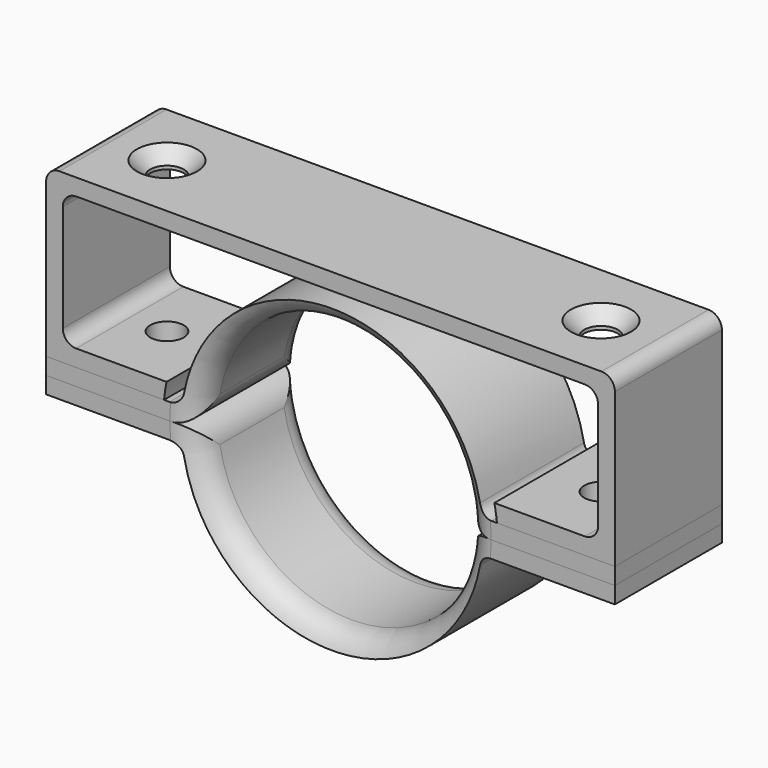
from build123d import *

# Parameters (mm, degrees)
F1_DEPTH      = 25.4
F2_DEPTH      = 25.4
F4_T1_DEPTH   = 48.6684264907
F4_T4_ANGLE   = 237.3879219603
F4_T6_ANGLE   = 237.3879219603
F4_2_T1_DEPTH = 48.6684264907
F4_2_T4_ANGLE = 237.3879219603
F4_2_T6_ANGLE = 237.3879219603
F5_R          = 2.54
F5_2_R        = 2.54
F6_W          = 3.175
F6_H          = 25.4
F7_DEPTH      = 25.4
F8_R          = 2.54
F3_R          = 3.175
F9_DEPTH      = 38.101
F10_SIZE      = 2.54
F10_2_SIZE    = 2.54


# Not quite as in the source:
# - a fillet or chamfer that OpenCascade refuses, or shapes differently, is made with other operations: its cross-section is extruded or revolved along the edge and cut away or added


with BuildPart() as f1:
    # F0 (on Front) → F1 (new body)
    with BuildSketch(Plane.XZ):
        with BuildLine():
            Line((-53.975, 0), (-28.575, 0))
            ThreePointArc((-28.575, 0), (-28.5307315382, 1.5899631749), (-28.3980633142, 3.175))
            Line((-28.3980633142, 3.175), (-53.975, 3.175))
            Line((-53.975, 3.175), (-53.975, 0))
        make_face()
        with BuildLine():
            Line((-28.575, 0), (-25.4, 0))
            ThreePointArc((-25.4, 0), (-25.3501463846, 1.5906219786), (-25.2007812379, 3.175))
            Line((-25.2007812379, 3.175), (-28.3980633142, 3.175))
            ThreePointArc((-28.3980633142, 3.175), (-28.5307315382, 1.5899631749), (-28.575, 0))
        make_face()
        with BuildLine():
            ThreePointArc((-25.2007812379, 3.175), (0, 25.4), (25.2007812379, 3.175))
            Line((25.2007812379, 3.175), (28.3980633142, 3.175))
            ThreePointArc((28.3980633142, 3.175), (0, 28.575), (-28.3980633142, 3.175))
            Line((-28.3980633142, 3.175), (-25.2007812379, 3.175))
        make_face()
        with BuildLine():
            ThreePointArc((25.2007812379, 3.175), (25.3501463846, 1.5906219786), (25.4, 0))
            Line((25.4, 0), (28.575, 0))
            ThreePointArc((28.575, 0), (28.5307315382, 1.5899631749), (28.3980633142, 3.175))
            Line((28.3980633142, 3.175), (25.2007812379, 3.175))
        make_face()
        with BuildLine():
            ThreePointArc((28.3980633142, 3.175), (28.5307315382, 1.5899631749), (28.575, 0))
            Line((28.575, 0), (53.975, 0))
            Line((53.975, 0), (53.975, 3.175))
            Line((53.975, 3.175), (28.3980633142, 3.175))
        make_face()
    extrude(amount=F1_DEPTH)

    # F4: fillet of radius 5.08 on 4 edges, made by hand

    # F4_s2 → F4_t1 (cut)
    with BuildSketch(Plane.XZ.offset(-11.6342132454)):
        with BuildLine():
            ThreePointArc((-30.0536852981, 0), (-26.7745593984, 1.2000859116), (-25.0447377485, 4.2333333333))
            ThreePointArc((-25.0447377485, 4.2333333333), (-25.3110286122, 2.1241070111), (-25.4, 0))
            Line((-25.4, 0), (-30.0536852981, 0))
        make_face()
        with BuildLine():
            ThreePointArc((25.0447377485, 4.2333333333), (26.7745593984, 1.2000859116), (30.0536852981, 0))
            Line((30.0536852981, 0), (25.4, 0))
            ThreePointArc((25.4, 0), (25.3110286122, 2.1241070111), (25.0447377485, 4.2333333333))
        make_face()
    extrude(amount=F4_T1_DEPTH, mode=Mode.SUBTRACT)

    # F4_s3 → F4_t4 (revolve, cut)
    with BuildSketch(Plane(origin=(0, 0, 0), x_dir=(0, 1, 0), z_dir=(0.4801310429, 0, -0.8771967748))):
        with BuildLine():
            ThreePointArc((-5.08, -25.4), (-1.4878975516, -26.8878975516), (0, -30.48))
            Line((0, -30.48), (0, -25.4))
            Line((0, -25.4), (-5.08, -25.4))
        make_face()
    revolve(axis=Axis((0, 0, 0), (0, 1, 0)), revolution_arc=F4_T4_ANGLE, mode=Mode.SUBTRACT)

    # F4_s5 → F4_t6 (revolve, cut)
    with BuildSketch(Plane(origin=(0, 0, 0), x_dir=(0, 1, 0), z_dir=(0.4801310429, 0, -0.8771967748))):
        with BuildLine():
            ThreePointArc((-20.32, -25.4), (-23.9121024484, -26.8878975516), (-25.4, -30.48))
            Line((-25.4, -30.48), (-25.4, -25.4))
            Line((-25.4, -25.4), (-20.32, -25.4))
        make_face()
    revolve(axis=Axis((0, -25.4, 0), (0, 1, 0)), revolution_arc=F4_T6_ANGLE, mode=Mode.SUBTRACT)

    # F5
    f5_edges = [f1.edges().sort_by_distance(p)[0] for p in [
        (-28.398063, -12.7, 3.175),
        (28.398063, -12.7, 3.175),
    ]]
    fillet(f5_edges, radius=F5_R)


with BuildPart() as f2:
    # F0 (on Front) → F2 (new body)
    with BuildSketch(Plane.XZ):
        with BuildLine():
            ThreePointArc((-28.3980633142, -3.175), (-28.5307315382, -1.5899631749), (-28.575, 0))
            Line((-28.575, 0), (-53.975, 0))
            Line((-53.975, 0), (-53.975, -3.175))
            Line((-53.975, -3.175), (-28.3980633142, -3.175))
        make_face()
        with BuildLine():
            ThreePointArc((-25.2007812379, -3.175), (-25.3501463846, -1.5906219786), (-25.4, 0))
            Line((-25.4, 0), (-28.575, 0))
            ThreePointArc((-28.575, 0), (-28.5307315382, -1.5899631749), (-28.3980633142, -3.175))
            Line((-28.3980633142, -3.175), (-25.2007812379, -3.175))
        make_face()
        with BuildLine():
            Line((28.3980633142, -3.175), (25.2007812379, -3.175))
            ThreePointArc((25.2007812379, -3.175), (0, -25.4), (-25.2007812379, -3.175))
            Line((-25.2007812379, -3.175), (-28.3980633142, -3.175))
            ThreePointArc((-28.3980633142, -3.175), (0, -28.575), (28.3980633142, -3.175))
        make_face()
        with BuildLine():
            Line((28.575, 0), (25.4, 0))
            ThreePointArc((25.4, 0), (25.3501463846, -1.5906219786), (25.2007812379, -3.175))
            Line((25.2007812379, -3.175), (28.3980633142, -3.175))
            ThreePointArc((28.3980633142, -3.175), (28.5307315382, -1.5899631749), (28.575, 0))
        make_face()
        with BuildLine():
            Line((53.975, 0), (28.575, 0))
            ThreePointArc((28.575, 0), (28.5307315382, -1.5899631749), (28.3980633142, -3.175))
            Line((28.3980633142, -3.175), (53.975, -3.175))
            Line((53.975, -3.175), (53.975, 0))
        make_face()
    extrude(amount=F2_DEPTH)

    # F4#2: fillet of radius 5.08 on 4 edges, made by hand

    # F4_2_s2 → F4_2_t1 (cut)
    with BuildSketch(Plane.XZ.offset(-11.6342132454)):
        with BuildLine():
            ThreePointArc((-25.0447377485, -4.2333333333), (-26.7745593984, -1.2000859116), (-30.0536852981, 0))
            Line((-30.0536852981, 0), (-25.4, 0))
            ThreePointArc((-25.4, 0), (-25.3110286122, -2.1241070111), (-25.0447377485, -4.2333333333))
        make_face()
        with BuildLine():
            ThreePointArc((30.0536852981, 0), (26.7745593984, -1.2000859116), (25.0447377485, -4.2333333333))
            ThreePointArc((25.0447377485, -4.2333333333), (25.3110286122, -2.1241070111), (25.4, 0))
            Line((25.4, 0), (30.0536852981, 0))
        make_face()
    extrude(amount=F4_2_T1_DEPTH, mode=Mode.SUBTRACT)

    # F4_2_s3 → F4_2_t4 (revolve, cut)
    with BuildSketch(Plane(origin=(0, 0, 0), x_dir=(0, 1, 0), z_dir=(-0.4801310429, 0, 0.8771967748))):
        with BuildLine():
            ThreePointArc((-5.08, -25.4), (-1.4878975516, -26.8878975516), (0, -30.48))
            Line((0, -30.48), (0, -25.4))
            Line((0, -25.4), (-5.08, -25.4))
        make_face()
    revolve(axis=Axis((0, 0, 0), (0, 1, 0)), revolution_arc=F4_2_T4_ANGLE, mode=Mode.SUBTRACT)

    # F4_2_s5 → F4_2_t6 (revolve, cut)
    with BuildSketch(Plane(origin=(0, 0, 0), x_dir=(0, 1, 0), z_dir=(-0.4801310429, 0, 0.8771967748))):
        with BuildLine():
            ThreePointArc((-20.32, -25.4), (-23.9121024484, -26.8878975516), (-25.4, -30.48))
            Line((-25.4, -30.48), (-25.4, -25.4))
            Line((-25.4, -25.4), (-20.32, -25.4))
        make_face()
    revolve(axis=Axis((0, -25.4, 0), (0, 1, 0)), revolution_arc=F4_2_T6_ANGLE, mode=Mode.SUBTRACT)

    # F5#2
    f5_2_edges = [f2.edges().sort_by_distance(p)[0] for p in [
        (-28.398063, -12.7, -3.175),
        (28.398063, -12.7, -3.175),
    ]]
    fillet(f5_2_edges, radius=F5_2_R)


with BuildPart() as f7:
    # F6 (on Front) → F7 (new body)
    with BuildSketch(Plane.XZ):
        with BuildLine():
            Line((-53.975, 3.175), (-31.5908511281, 3.175))
            ThreePointArc((-31.5908511281, 3.175), (-31.3898539795, 4.7686022212), (-31.1085197333, 6.35))
            Line((-31.1085197333, 6.35), (-50.8, 6.35))
            Line((-50.8, 6.35), (-53.975, 6.35))
            Line((-53.975, 6.35), (-53.975, 3.175))
        make_face()
        with Locations((-52.3875, 19.05)):
            Rectangle(F6_W, F6_H)
        Polygon((-50.8, 31.75), (7.66e-08, 31.75), (50.8, 31.75), (53.975, 31.75), (53.975, 34.925), (-53.975, 34.925), (-53.975, 31.75), align=None)
        with Locations((52.3875, 19.05)):
            Rectangle(F6_W, F6_H)
        with BuildLine():
            ThreePointArc((31.1085197333, 6.35), (31.3898539795, 4.7686022212), (31.5908511281, 3.175))
            Line((31.5908511281, 3.175), (53.975, 3.175))
            Line((53.975, 3.175), (53.975, 6.35))
            Line((53.975, 6.35), (50.8, 6.35))
            Line((50.8, 6.35), (31.1085197333, 6.35))
        make_face()
    extrude(amount=F7_DEPTH)

    # F8
    f8_edges = [f7.edges().sort_by_distance(p)[0] for p in [
        (-50.8, -12.7, 6.35),
        (50.8, -12.7, 6.35),
        (50.8, -12.7, 31.75),
        (-50.8, -12.7, 31.75),
        (53.975, -12.7, 34.925),
        (-53.975, -12.7, 34.925),
    ]]
    fillet(f8_edges, radius=F8_R)


with BuildPart() as f9_tool:
    # F3 (on face) → F9 (new body, through all)
    with BuildSketch(Plane(origin=(0, 0, -3.175), x_dir=(1, 0, 0), z_dir=(0, 0, -1))):
        with Locations((-41.1865316571, 12.7)):
            Circle(F3_R)
        with Locations((41.1865316571, 12.7)):
            Circle(F3_R)
    extrude(amount=-F9_DEPTH)


with BuildPart() as f1_1:
    add(f1.part)

    # F9: cut by f9_tool
    add(f9_tool.part, mode=Mode.SUBTRACT)


with BuildPart() as f2_1:
    add(f2.part)

    # F9: cut by f9_tool
    add(f9_tool.part, mode=Mode.SUBTRACT)

    # F10#2
    f10_2_edges = [f2_1.edges().sort_by_distance(p)[0] for p in [
        (-44.361532, -12.7, -3.175),
        (38.011532, -12.7, -3.175),
    ]]
    chamfer(f10_2_edges, length=F10_2_SIZE)


with BuildPart() as f7_1:
    add(f7.part)

    # F9: cut by f9_tool
    add(f9_tool.part, mode=Mode.SUBTRACT)

    # F10
    f10_edges = [f7_1.edges().sort_by_distance(p)[0] for p in [
        (-44.361532, -12.7, 34.925),
        (38.011532, -12.7, 34.925),
    ]]
    chamfer(f10_edges, length=F10_SIZE)


solid = Compound([f1_1.part, f2_1.part, f7_1.part])
